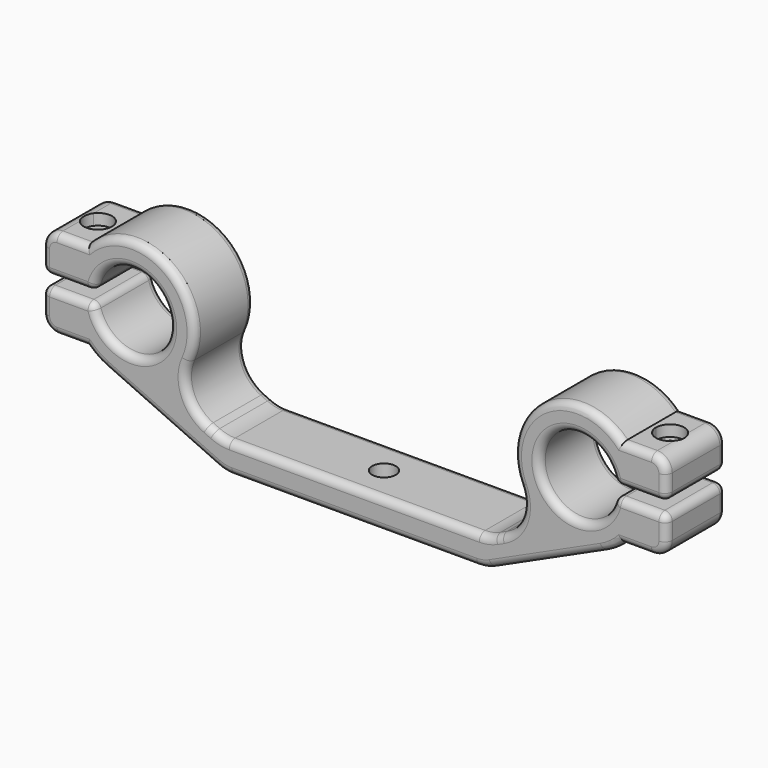
from build123d import *

# Parameters (mm, degrees)
F1_DEPTH  = 5
F2_R      = 2
F3_R      = 5
F4_R      = 1.05
F5_DEPTH  = 1.5
F6_DEPTH  = 14.501
F7_R      = 1.05
F8_DEPTH  = 1.5
F9_R      = 1
F11_R     = 1.6
F12_DEPTH = 23.501
F13_R     = 1


# Not quite as in the source:
# - a feature names something its author has since deleted; it is built from what else it names


with BuildPart() as f1:
    # F0 (on Front) → F1 (new body, symmetric)
    with BuildSketch(Plane.XZ):
        with BuildLine():
            ThreePointArc((-35.0445515162, 0.75), (-24.9, 0), (-35.0445515162, -0.75))
            Line((-35.0445515162, -0.75), (-42, -0.75))
            Line((-42, -0.75), (-42, -6))
            Line((-42, -6), (-36.0207972894, -6))
            ThreePointArc((-36.0207972894, -6), (-34.84999119, -6.9805146986), (-33.5226296575, -7.735701668))
            Line((-33.5226296575, -7.735701668), (-17.5702162087, -15))
            Line((-17.5702162087, -15), (0, -15))
            Line((0, -15), (0, -11))
            Line((0, -11), (-17.908828776, -11))
            Line((-17.908828776, -11), (-25.8163518373, -7.3991275196))
            ThreePointArc((-25.8163518373, -7.3991275196), (-23.237756748, 5.1499578834), (-36.0207972894, 6))
            Line((-36.0207972894, 6), (-42, 6))
            Line((-42, 6), (-42, 0.75))
            Line((-42, 0.75), (-35.0445515162, 0.75))
        make_face()
    extrude(amount=F1_DEPTH, both=True)

    # F2
    f2_edges = [f1.edges().sort_by_distance(p)[0] for p in [
        (-42, 0, 6),
        (-42, 0, -6),
    ]]
    fillet(f2_edges, radius=F2_R)

    # F3
    f3_edges = [f1.edges().sort_by_distance(p)[0] for p in [
        (-25.816352, 0, -7.399128),
        (-17.908829, 0, -11),
        (-17.570216, 0, -15),
    ]]
    fillet(f3_edges, radius=F3_R)

    # F4 (on face) → F5 (cut, symmetric)
    with BuildSketch(Plane(origin=(0, 0, -6), x_dir=(1, 0, 0), z_dir=(0, 0, -1))):
        Polygon((-36.5, -1.1547005384), (-36.5, 1.1547005384), (-38.5, 2.3094010768), (-40, 1.443375673), (-40, -1.443375673), (-38.5, -2.3094010768), align=None)
        with Locations((-38.5, 0)):
            Circle(F4_R, mode=Mode.SUBTRACT)
        Polygon((-40, -1.443375673), (-40, 1.443375673), (-40.5, 1.1547005384), (-40.5, -1.1547005384), align=None)
    extrude(amount=F5_DEPTH, both=True, mode=Mode.SUBTRACT)

    # F6 (cut, through all): a face of the model
    f6_faces = [f1.faces().sort_by_distance(p)[0] for p in [
        (-38.5, 0, -6),
    ]]
    extrude(f6_faces, amount=-F6_DEPTH, mode=Mode.SUBTRACT)

    # F7 (on face) → F8 (cut, symmetric)
    with BuildSketch(Plane.XY.offset(6)):
        with BuildLine():
            ThreePointArc((-40, -1.166190379), (-37.8835585997, -1.7972200756), (-36.6, 0))
            ThreePointArc((-36.6, 0), (-37.8835585997, 1.7972200756), (-40, 1.166190379))
            Line((-40, 1.166190379), (-40, -1.166190379))
        make_face()
        with Locations((-38.5, 0)):
            Circle(F7_R, mode=Mode.SUBTRACT)
        with Locations((-38.5, 0)):
            Circle(F7_R)
        with BuildLine():
            Line((-40, -1.166190379), (-40, 1.166190379))
            ThreePointArc((-40, 1.166190379), (-40.4, 0), (-40, -1.166190379))
        make_face()
    extrude(amount=F8_DEPTH, both=True, mode=Mode.SUBTRACT)

    # F9
    f9_edges = [f1.edges().sort_by_distance(p)[0] for p in [
        (-35.044552, 0, -0.75),
        (-35.044552, 0, 0.75),
    ]]
    fillet(f9_edges, radius=F9_R)

    # F10: F1 across plane


with BuildPart() as f1_1:
    add(f1.part)
    add(f1.part.mirror(Plane.YZ))

    # F11 (on face) → F12 (cut, through all)
    with BuildSketch(Plane(origin=(0, 0, -15), x_dir=(1, 0, 0), z_dir=(0, 0, -1))):
        Circle(F11_R)
    extrude(amount=-F12_DEPTH, mode=Mode.SUBTRACT)

    # F13
    f13_edges = [f1_1.edges().sort_by_distance(p)[0] for p in [
        (0, -5, -11),
        (0, -5, -15),
        (-24.9, -5, 0),
        (24.9, -5, 0),
        (42, -5, 2.375),
        (42, -5, -2.375),
        (-42, -5, -2.375),
        (-42, -5, 2.375),
        (-42, 5, 2.375),
        (-42, 5, -2.375),
        (-38.921793, 5, -0.75),
        (-26.04007, 5, -11.143057),
        (-22.396734, 5, -7.347172),
        (42, 5, 2.375),
        (38.921793, 5, 0.75),
        (42, 5, -2.375),
        (42, 0, -0.75),
        (42, 0, 0.75),
        (-42, 0, 0.75),
        (-42, 0, -0.75),
        (-38.921793, 5, 0.75),
        (-35.246462, 5, 0.947851),
        (-24.9, 5, 0),
        (-35.246462, 5, -0.947851),
        (-41.414214, 5, -5.414214),
        (-38.010399, 5, -6),
        (-34.849991, 5, -6.980515),
        (-17.545549, 5, -14.886311),
        (0, 5, -15),
        (17.545549, 5, -14.886311),
        (26.04007, 5, -11.143057),
        (34.849991, 5, -6.980515),
        (38.010399, 5, -6),
        (41.414214, 5, -5.414214),
        (38.921793, 5, -0.75),
        (35.246462, 5, -0.947851),
        (24.9, 5, 0),
        (35.246462, 5, 0.947851),
        (41.414214, 5, 5.414214),
        (38.010399, 5, 6),
        (25.162093, 5, 6.988895),
        (22.396734, 5, -7.347172),
        (19.341072, 5, -10.347795),
        (17.884162, 5, -10.886311),
        (0, 5, -11),
        (-17.884162, 5, -10.886311),
        (-19.341072, 5, -10.347795),
        (-25.162093, 5, 6.988895),
        (-38.010399, 5, 6),
        (-41.414214, 5, 5.414214),
        (-38.921793, -5, 0.75),
        (-35.246462, -5, 0.947851),
        (-35.246462, -5, -0.947851),
        (-38.921793, -5, -0.75),
        (-41.414214, -5, -5.414214),
        (-38.010399, -5, -6),
        (-34.849991, -5, -6.980515),
        (-26.04007, -5, -11.143057),
        (-17.545549, -5, -14.886311),
        (17.545549, -5, -14.886311),
        (26.04007, -5, -11.143057),
        (34.849991, -5, -6.980515),
        (38.010399, -5, -6),
        (41.414214, -5, -5.414214),
        (38.921793, -5, -0.75),
        (35.246462, -5, -0.947851),
        (35.246462, -5, 0.947851),
        (38.921793, -5, 0.75),
        (41.414214, -5, 5.414214),
        (38.010399, -5, 6),
        (25.162093, -5, 6.988895),
        (22.396734, -5, -7.347172),
        (19.341072, -5, -10.347795),
        (17.884162, -5, -10.886311),
        (-17.884162, -5, -10.886311),
        (-19.341072, -5, -10.347795),
        (-22.396734, -5, -7.347172),
        (-25.162093, -5, 6.988895),
        (-38.010399, -5, 6),
        (-41.414214, -5, 5.414214),
    ]]
    fillet(f13_edges, radius=F13_R)


solid = f1_1.part
